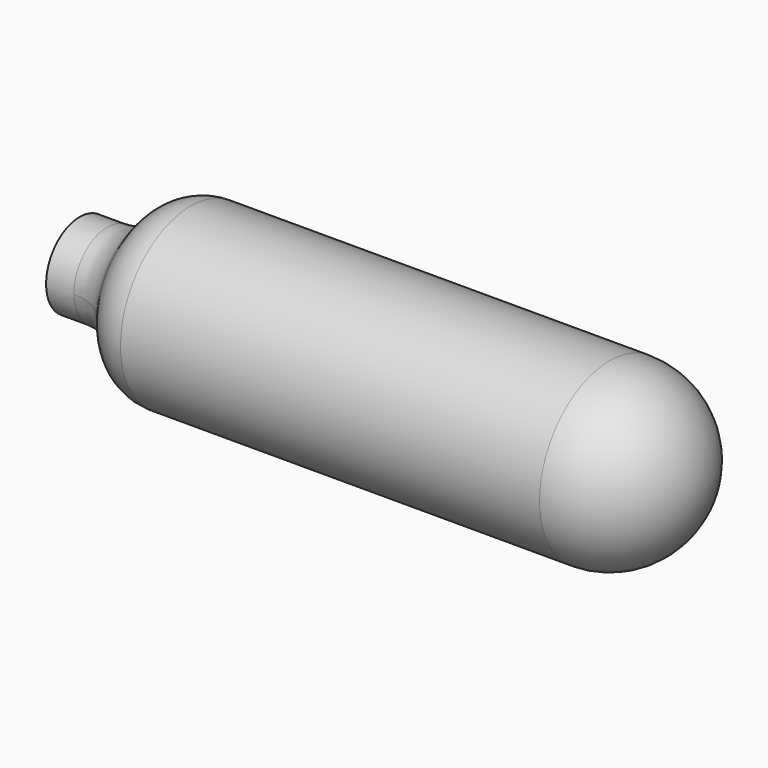
from build123d import *

# Parameters (mm, degrees)
F0_R     = 9.017
F1_DEPTH = 57.15
F2_R     = 4.318
F3_DEPTH = 6.35
F5_R     = 9.017
F7_R     = 5.08


# Not quite as in the source:
# - a fillet or chamfer that OpenCascade refuses, or shapes differently, is made with other operations: its cross-section is extruded or revolved along the edge and cut away or added


with BuildPart() as f1:
    # F0 (on Right) → F1 (new body)
    with BuildSketch(Plane.YZ):
        Circle(F0_R)
    extrude(amount=F1_DEPTH)

    # F2 (on face) → F3 (join)
    with BuildSketch(Plane(origin=(0, 0, 0), x_dir=(0, -1, 0), z_dir=(-1, 0, 0))):
        Circle(F2_R)
    extrude(amount=F3_DEPTH)

    # F5
    f5_edges = [f1.edges().sort_by_distance(p)[0] for p in [
        (57.15, -9.017, 0),
    ]]
    fillet(f5_edges, radius=F5_R)

    # F6: fillet of radius 5.08 on 3 edges, made by hand

    # F6_s1 → F6_t2 (revolve, cut)
    with BuildSketch(Plane.XY):
        with BuildLine():
            ThreePointArc((5.0656923515, 9.017), (1.6109188423, 7.6613710878), (0, 4.318))
            Line((0, 4.318), (0, 9.017))
            Line((0, 9.017), (5.0656923515, 9.017))
        make_face()
    revolve(axis=Axis((0, 0, 0), (1, 0, 0)), mode=Mode.SUBTRACT)

    # F7
    f7_edges = [f1.edges().sort_by_distance(p)[0] for p in [
        (0, 0, 4.318),
        (0, 0, -4.318),
    ]]
    fillet(f7_edges, radius=F7_R)


solid = f1.part
